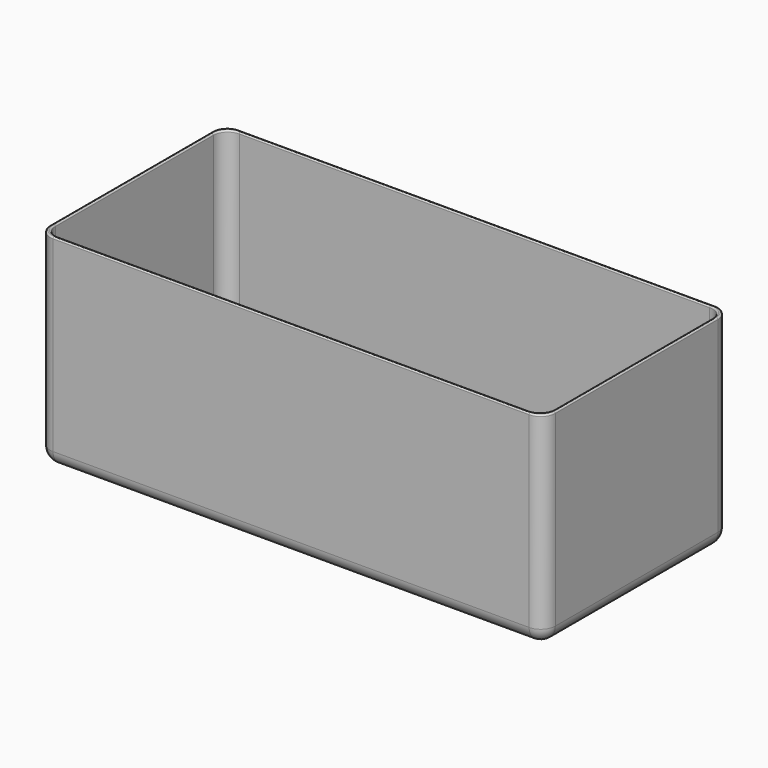
from build123d import *

# Parameters (mm, degrees)
F0_W     = 174
F0_H     = 80
F1_DEPTH = 70
F2_W     = 172
F2_H     = 78
F3_DEPTH = 69
F4_R     = 5
F5_R     = 5
F6_R     = 0.49999


# Not quite as in the source:
# - a fillet or chamfer is up to 0.001 mm smaller than in the source, because OpenCascade refuses the exact size


with BuildPart() as f1:
    # F0 (on Top) → F1 (new body)
    with BuildSketch(Plane.XY):
        Rectangle(F0_W, F0_H)
    extrude(amount=F1_DEPTH)

    # F2 (on face) → F3 (cut)
    with BuildSketch(Plane.XY.offset(70)):
        Rectangle(F2_W, F2_H)
    extrude(amount=-F3_DEPTH, mode=Mode.SUBTRACT)

    # F4
    f4_edges = [f1.edges().sort_by_distance(p)[0] for p in [
        (-86, 39, 35.5),
        (-86, -39, 35.5),
        (86, -39, 35.5),
        (86, 39, 35.5),
        (0, -39, 1),
        (86, 0, 1),
        (0, 39, 1),
        (-86, 0, 1),
        (0, -40, 0),
    ]]
    fillet(f4_edges, radius=F4_R)

    # F5
    f5_edges = [f1.edges().sort_by_distance(p)[0] for p in [
        (0, -40, 5),
        (-87, -40, 37.5),
        (-87, 40, 35),
        (87, 2.5, 0),
        (87, 40, 35),
        (0, 40, 0),
    ]]
    fillet(f5_edges, radius=F5_R)

    # F6 (radius 0.5 in the source; OpenCascade refuses exactly that, so slightly less here)
    f6_edges = [f1.edges().sort_by_distance(p)[0] for p in [
        (0, 40, 70),
        (0, -39, 70),
        (0, 39, 70),
        (86, 0, 70),
        (-84.535534, -37.535534, 70),
        (-86, 0, 70),
        (84.535534, 37.535534, 70),
        (0, -40, 70),
        (87, 0, 70),
        (85.535534, -38.535534, 70),
        (-87, 0, 70),
        (-85.535534, -38.535534, 70),
        (-85.535534, 38.535534, 70),
        (85.535534, 38.535534, 70),
        (84.535534, -37.535534, 70),
        (-84.535534, 37.535534, 70),
    ]]
    fillet(f6_edges, radius=F6_R)


solid = f1.part
